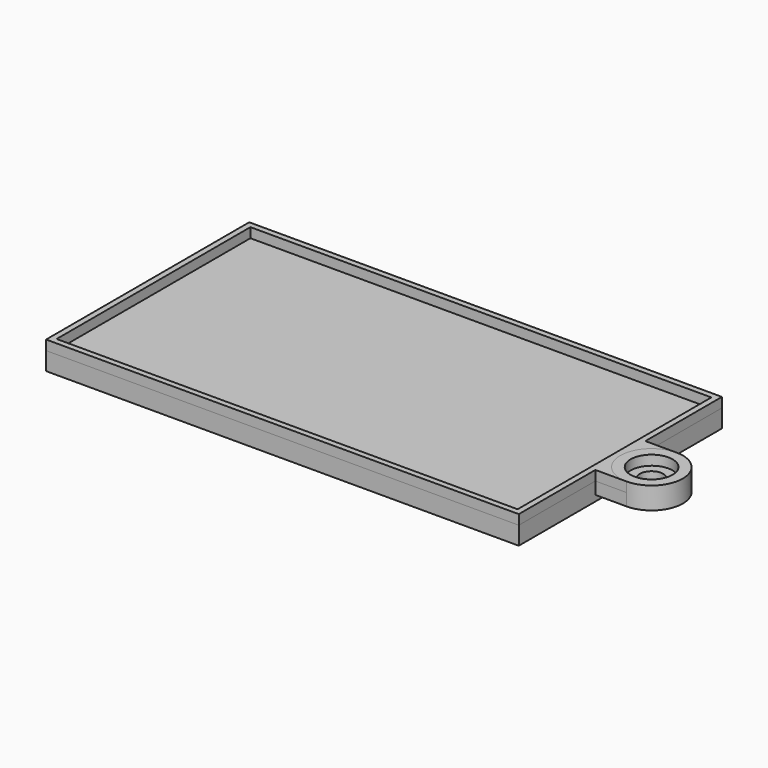
from build123d import *

# Parameters (mm, degrees)
F1_DEPTH  = 1.5875
F2_R      = 1.524
F3_DEPTH  = 1.5885
F4_R      = 2.7305
F5_DEPTH  = 1.27
F6_W      = 1.524
F6_H      = 6.35
F7_DEPTH  = 1.524
F8_W      = 6.35
F8_H      = 0.508
F9_DEPTH  = 1.016
F10_SIZE  = 0.50799
F12_DEPTH = 0.762
F13_W     = 59.944
F13_H     = 31.496
F14_DEPTH = 1.27
F15_W     = 45.72
F15_H     = 1.524
F16_DEPTH = 0.762


# Not quite as in the source:
# - a fillet or chamfer is up to 0.001 mm smaller than in the source, because OpenCascade refuses the exact size
# - a pattern or mirror of a feature is missing from the dataset's text; its kind, count and spacing are read off the source's solid


with BuildPart() as f1:
    # F0 (on Top) → F1 (new body)
    with BuildSketch(Plane.XY):
        Polygon((-30.734, -16.51), (30.734, -16.51), (30.734, -4.064), (30.734, 4.064), (30.734, 16.51), (-30.734, 16.51), align=None)
        with BuildLine():
            Line((30.734, 4.064), (30.734, -4.064))
            Line((30.734, -4.064), (34.798, -4.064))
            ThreePointArc((34.798, -4.064), (37.6716819587, -2.8736819587), (38.862, 0))
            ThreePointArc((38.862, 0), (37.6716819587, 2.8736819587), (34.798, 4.064))
            Line((34.798, 4.064), (30.734, 4.064))
        make_face()
    extrude(amount=F1_DEPTH)

    # F2 (on face) → F3 (cut, through all)
    with BuildSketch(Plane.XY.offset(1.5875)):
        with Locations((34.798, 0)):
            Circle(F2_R)
    extrude(amount=-F3_DEPTH, mode=Mode.SUBTRACT)

    # F4 (on face) → F5 (join)
    with BuildSketch(Plane.XY.offset(1.5875)):
        with BuildLine():
            ThreePointArc((34.798, -4.064), (37.6716819587, -2.8736819587), (38.862, 0))
            ThreePointArc((38.862, 0), (37.6716819587, 2.8736819587), (34.798, 4.064))
            ThreePointArc((34.798, 4.064), (30.734, 0), (34.798, -4.064))
        make_face()
        with Locations((34.798, 0)):
            Circle(F4_R, mode=Mode.SUBTRACT)
    extrude(amount=F5_DEPTH)

    # F6 (on face) → F7 (join)
    with BuildSketch(Plane(origin=(0, 0, 0), x_dir=(1, 0, 0), z_dir=(0, 0, -1))):
        with Locations((-29.972, 0)):
            Rectangle(F6_W, F6_H)
    extrude(amount=F7_DEPTH)

    # F8 (on face) → F9 (join)
    with BuildSketch(Plane(origin=(-30.734, 0, 0), x_dir=(0, -1, 0), z_dir=(-1, 0, 0))):
        with Locations((0, -1.27)):
            Rectangle(F8_W, F8_H)
    extrude(amount=F9_DEPTH)

    # F10 (size 0.508 in the source; OpenCascade refuses exactly that, so slightly less here)
    f10_edges = [f1.edges().sort_by_distance(p)[0] for p in [
        (-31.75, 0, -1.016),
        (-29.21, 0, -1.524),
    ]]
    chamfer(f10_edges, length=F10_SIZE)

    # F11 (on face) → F12 (join)
    with BuildSketch(Plane(origin=(0, 0, 0), x_dir=(1, 0, 0), z_dir=(0, 0, -1))):
        Polygon((-29.972, 3.175), (-29.972, 15.748), (29.972, 15.748), (29.972, -15.748), (-29.972, -15.748), (-29.972, -3.175), (-30.734, -3.175), (-30.734, -16.51), (30.734, -16.51), (30.734, -4.064), (30.734, 4.064), (30.734, 16.51), (-30.734, 16.51), (-30.734, 3.175), align=None)
    extrude(amount=F12_DEPTH)

    # F13 (on face) → F14 (join, through all)
    with BuildSketch(Plane.XY.offset(1.5875)):
        with BuildLine():
            ThreePointArc((34.798, -4.064), (31.9243180414, -2.8736819589), (30.734, -4e-10))
            Line((30.734, -4e-10), (30.734, -4.064))
            Line((30.734, -4.064), (34.798, -4.064))
        make_face()
        with BuildLine():
            Line((34.798, 4.064), (30.734, 4.064))
            Line((30.734, 4.064), (30.734, -4e-10))
            ThreePointArc((30.734, -4e-10), (31.9243180411, 2.8736819586), (34.798, 4.064))
        make_face()
        Polygon((30.734, 16.51), (-30.734, 16.51), (-30.734, -16.51), (30.734, -16.51), (30.734, -4.064), (30.734, -4e-10), (30.734, 4.064), align=None)
        Rectangle(F13_W, F13_H, mode=Mode.SUBTRACT)
    extrude(amount=F14_DEPTH)

    # F15 (on face) → F16 (join)
    with BuildSketch(Plane(origin=(0, 0, 0), x_dir=(1, 0, 0), z_dir=(0, 0, -1))):
        with Locations((0, 7.874)):
            Rectangle(F15_W, F15_H)
    f16 = extrude(amount=F16_DEPTH)

    # F16_copies: F16 across plane
    add(f16.mirror(Plane.ZX))


solid = f1.part
